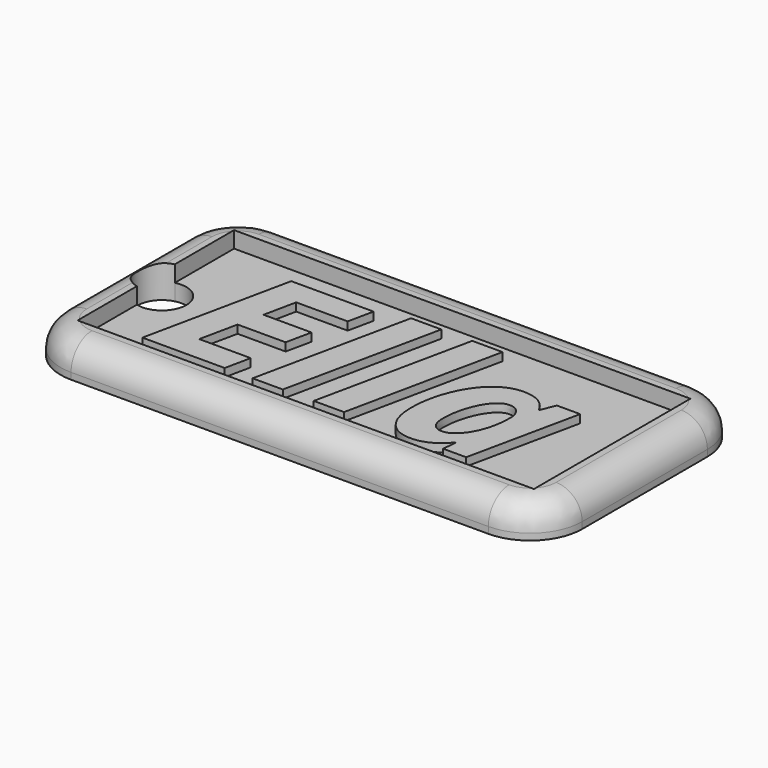
from build123d import *

# Parameters (mm, degrees)
F1_DEPTH     = 1.5875
F0_W         = 50.8
F0_H         = 25.4
F2_DEPTH     = 3.175
F3_R         = 5.08
F4_T1_DEPTH  = 40.64
F4_T3_DEPTH  = 15.24
F4_T6_ANGLE  = 90
F4_T8_ANGLE  = 90
F4_T10_ANGLE = 90
F4_T12_ANGLE = 90
F5_TEXT_SIZE = 20.0745287455
F6_DEPTH     = 0.79375


# Not quite as in the source:
# - a fillet or chamfer that OpenCascade refuses, or shapes differently, is made with other operations: its cross-section is extruded or revolved along the edge and cut away or added
# - Text() gives the source's letters only with a copy of the font that has no kerning and outlines rounded to 1/6400 em; it was checked with that copy


with BuildPart() as f1:
    # F0 (on Top) → F1 (new body)
    with BuildSketch(Plane.XY):
        with BuildLine():
            ThreePointArc((3.175, 15.0070376392), (5.2252931644, 14.5808168074), (6.1461049769, 12.7))
            ThreePointArc((6.1461049769, 12.7), (5.2252931644, 10.8191831926), (3.175, 10.3929623608))
            Line((3.175, 10.3929623608), (3.175, 3.175))
            Line((3.175, 3.175), (47.625, 3.175))
            Line((47.625, 3.175), (47.625, 22.225))
            Line((47.625, 22.225), (3.175, 22.225))
            Line((3.175, 22.225), (3.175, 15.0070376392))
        make_face()
    extrude(amount=F1_DEPTH)

    # F0 (on Top) → F2 (join)
    with BuildSketch(Plane.XY):
        with Locations((25.4, 12.7)):
            Rectangle(F0_W, F0_H)
        with BuildLine():
            ThreePointArc((3.175, 10.3929623608), (1.3836049769, 12.7), (3.175, 15.0070376392))
            Line((3.175, 15.0070376392), (3.175, 22.225))
            Line((3.175, 22.225), (47.625, 22.225))
            Line((47.625, 22.225), (47.625, 3.175))
            Line((47.625, 3.175), (3.175, 3.175))
            Line((3.175, 3.175), (3.175, 10.3929623608))
        make_face(mode=Mode.SUBTRACT)
    extrude(amount=F2_DEPTH)

    # F3
    f3_edges = [f1.edges().sort_by_distance(p)[0] for p in [
        (0, 0, 1.5875),
        (50.8, 0, 1.5875),
        (50.8, 25.4, 1.5875),
        (0, 25.4, 1.5875),
    ]]
    fillet(f3_edges, radius=F3_R)

    # F4: fillet of radius 2.54 on 8 edges, made by hand

    # F4_s2 → F4_t1 (cut)
    with BuildSketch(Plane.YZ.offset(5.08)):
        with BuildLine():
            ThreePointArc((22.86, 3.175), (24.6560512242, 2.4310512242), (25.4, 0.635))
            Line((25.4, 0.635), (25.4, 3.175))
            Line((25.4, 3.175), (22.86, 3.175))
        make_face()
        with BuildLine():
            ThreePointArc((2.54, 3.175), (0.7439487758, 2.4310512242), (0, 0.635))
            Line((0, 0.635), (0, 3.175))
            Line((0, 3.175), (2.54, 3.175))
        make_face()
    extrude(amount=F4_T1_DEPTH, mode=Mode.SUBTRACT)

    # F4_s4 → F4_t3 (cut)
    with BuildSketch(Plane.XZ.offset(-20.32)):
        with BuildLine():
            ThreePointArc((2.54, 3.175), (0.7439487758, 2.4310512242), (0, 0.635))
            Line((0, 0.635), (0, 3.175))
            Line((0, 3.175), (2.54, 3.175))
        make_face()
        with BuildLine():
            ThreePointArc((48.26, 3.175), (50.0560512242, 2.4310512242), (50.8, 0.635))
            Line((50.8, 0.635), (50.8, 3.175))
            Line((50.8, 3.175), (48.26, 3.175))
        make_face()
    extrude(amount=F4_T3_DEPTH, mode=Mode.SUBTRACT)

    # F4_s5 → F4_t6 (revolve, cut)
    with BuildSketch(Plane.YZ.offset(5.08)):
        with BuildLine():
            ThreePointArc((22.86, 3.175), (24.6560512242, 2.4310512242), (25.4, 0.635))
            Line((25.4, 0.635), (25.4, 3.175))
            Line((25.4, 3.175), (22.86, 3.175))
        make_face()
    revolve(axis=Axis((5.08, 20.32, 3.175), (0, 0, 1)), revolution_arc=F4_T6_ANGLE, mode=Mode.SUBTRACT)

    # F4_s7 → F4_t8 (revolve, cut)
    with BuildSketch(Plane.YZ.offset(5.08)):
        with BuildLine():
            ThreePointArc((2.54, 3.175), (0.7439487758, 2.4310512242), (0, 0.635))
            Line((0, 0.635), (0, 3.175))
            Line((0, 3.175), (2.54, 3.175))
        make_face()
    revolve(axis=Axis((5.08, 5.08, 3.175), (0, 0, -1)), revolution_arc=F4_T8_ANGLE, mode=Mode.SUBTRACT)

    # F4_s9 → F4_t10 (revolve, cut)
    with BuildSketch(Plane.YZ.offset(45.72)):
        with BuildLine():
            ThreePointArc((22.86, 3.175), (24.6560512242, 2.4310512242), (25.4, 0.635))
            Line((25.4, 0.635), (25.4, 3.175))
            Line((25.4, 3.175), (22.86, 3.175))
        make_face()
    revolve(axis=Axis((45.72, 20.32, 3.175), (0, 0, -1)), revolution_arc=F4_T10_ANGLE, mode=Mode.SUBTRACT)

    # F4_s11 → F4_t12 (revolve, cut)
    with BuildSketch(Plane.XZ.offset(-5.08)):
        with BuildLine():
            ThreePointArc((48.26, 3.175), (50.0560512242, 2.4310512242), (50.8, 0.635))
            Line((50.8, 0.635), (50.8, 3.175))
            Line((50.8, 3.175), (48.26, 3.175))
        make_face()
    revolve(axis=Axis((45.72, 5.08, 3.175), (0, 0, -1)), revolution_arc=F4_T12_ANGLE, mode=Mode.SUBTRACT)

    # F5 (on face) → F6 (join)
    with BuildSketch(Plane.XY.offset(1.5875)):
        with Locations((7.3244902305, 5.2343793213)):
            Text('Ella', F5_TEXT_SIZE, font='Open Sans', font_style=FontStyle.BOLDITALIC, text_align=(TextAlign.LEFT, TextAlign.BOTTOM))
    extrude(amount=F6_DEPTH)


solid = f1.part
